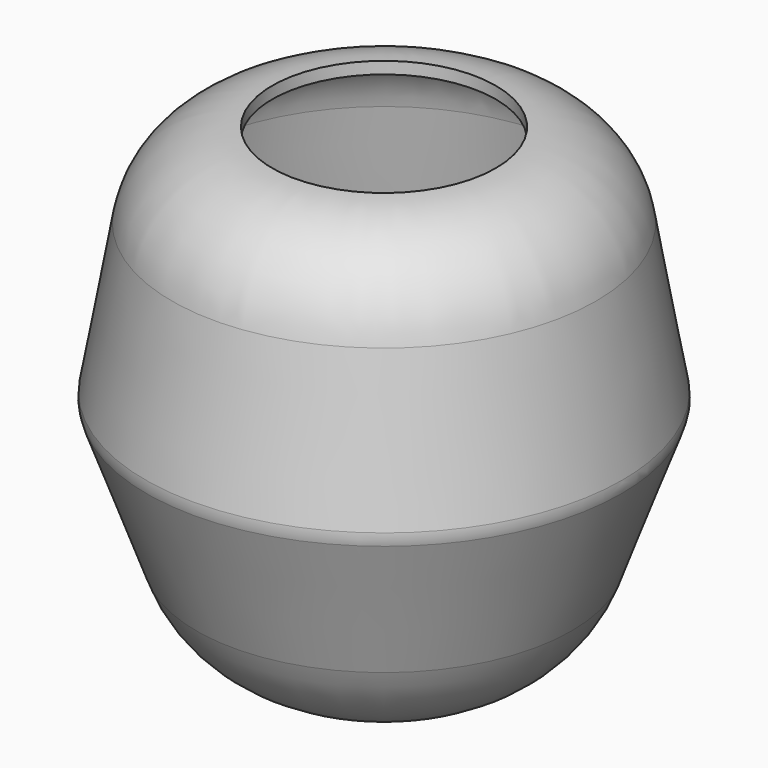
from build123d import *

# Parameters (mm, degrees)
F0_R          = 50.8
F1_DEPTH      = 50.8
F1_TAPER      = 10
F1_DEPTH_BACK = 50.8
F1_TAPER_BACK = 20
F2_R          = 5.08
F3_R          = 31.0633576014
F4_R          = 21.6235834267
F5_T          = -2.54


# Not quite as in the source:
# - a shell that OpenCascade refuses in one call is made with other operations: the cavity is built on its own and cut out


with BuildPart() as f1:
    # F0 (on Top) → F1 (new body, two sides)
    with BuildSketch(Plane.XY) as f1_sk:
        Circle(F0_R)
    extrude(amount=F1_DEPTH, taper=F1_TAPER)
    extrude(f1_sk.sketch, amount=-F1_DEPTH_BACK, taper=F1_TAPER_BACK)

    # F2
    f2_edges = [f1.edges().sort_by_distance(p)[0] for p in [
        (-50.8, 0, 0),
    ]]
    fillet(f2_edges, radius=F2_R)

    # F3
    f3_edges = [f1.edges().sort_by_distance(p)[0] for p in [
        (-32.310312, 0, -50.8),
    ]]
    fillet(f3_edges, radius=F3_R)

    # F4
    f4_edges = [f1.edges().sort_by_distance(p)[0] for p in [
        (-41.842589, 0, 50.8),
    ]]
    fillet(f4_edges, radius=F4_R)

    # F5: a shell. OpenCascade refuses it in one call, so the cavity is built on its own and cut out:
    # the body offset inwards by the wall thickness, plus a prism from it out through each open face.
    f5_core = offset(f1.part, amount=F5_T, mode=Mode.PRIVATE)
    f5_exits = [f5_core.faces().sort_by_distance(p)[0] for p in [
        (0, 0, 48.26),
    ]]
    add(f5_core, mode=Mode.SUBTRACT)
    extrude(f5_exits, amount=-F5_T, mode=Mode.SUBTRACT)


solid = f1.part
